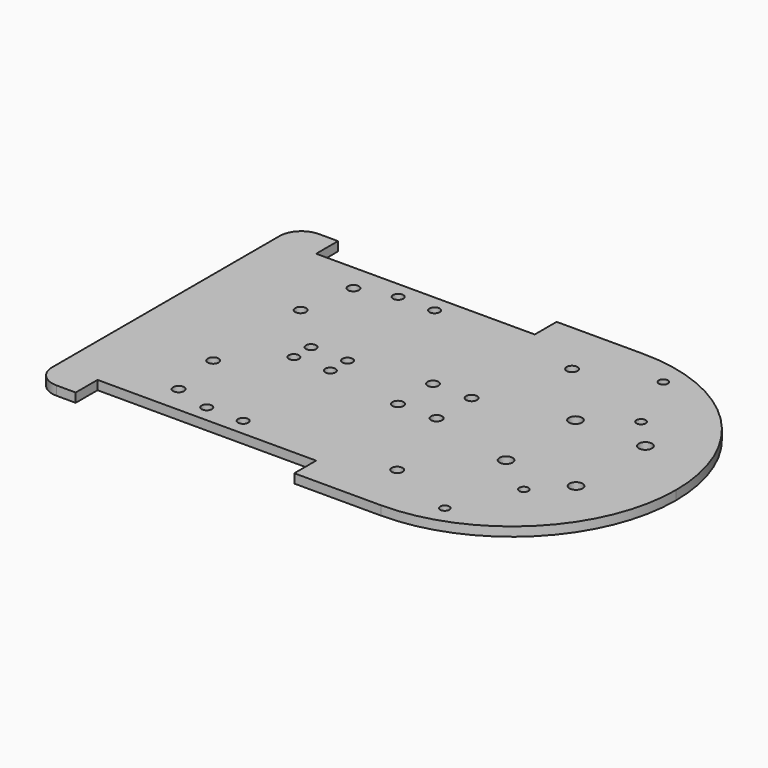
from build123d import *

# Parameters (mm, degrees)
F0_W     = 177.8
F0_H     = 114.3
F1_DEPTH = 3.175
F2_R     = 7.62
F3_W     = 76.2
F3_H     = 9.525
F4_DEPTH = 25.4
F6_D     = 3.556
F8_D     = 3.81
F11_D    = 3.81
F13_D    = 4.572
F15_D    = 3.81
F16_R    = 57.14999
F18_D    = 3.175


# Not quite as in the source:
# - a fillet or chamfer is up to 0.001 mm smaller than in the source, because OpenCascade refuses the exact size


with BuildPart() as f1:
    # F0 (on Top) → F1 (new body)
    with BuildSketch(Plane.XY):
        with Locations((34.6569041669, 50.5347196277)):
            Rectangle(F0_W, F0_H)
    extrude(amount=F1_DEPTH)

    # F2
    f2_edges = [f1.edges().sort_by_distance(p)[0] for p in [
        (-54.243096, 107.68472, 1.5875),
        (-54.243096, -6.61528, 1.5875),
    ]]
    fillet(f2_edges, radius=F2_R)

    # F3 (on face) → F4 (cut)
    with BuildSketch(Plane.XY.offset(3.175)):
        with Locations((-1.8555958331, -1.8527803723)):
            Rectangle(F3_W, F3_H)
        with Locations((-1.8555958331, 102.9222196277)):
            Rectangle(F3_W, F3_H)
    extrude(amount=-F4_DEPTH, mode=Mode.SUBTRACT)

    # F6 (through all)
    with Locations(Plane.XY.offset(3.175)):
        with Locations((-6.6180958331, 8.8279196277), (-6.6180958331, 46.7755196277), (-6.6180958331, 54.2939196277), (-6.6180958331, 92.2415196277), (6.0819041669, 8.8279196277), (6.0819041669, 46.7755196277), (6.0819041669, 54.2939196277), (6.0819041669, 92.2415196277)):
            Hole(F6_D / 2)

    # F8 (through all)
    with Locations(Plane.XY.offset(3.175)):
        with Locations((32.7773041669, 42.9147196277), (46.2393041669, 42.9147196277), (46.2393041669, 58.1547196277), (32.7773041669, 58.1547196277)):
            Hole(F8_D / 2)

    # F11 (through all)
    with Locations(Plane.XY.offset(3.175)):
        with Locations((-22.4930958331, 31.4847196277), (-22.4930958331, 69.5847196277)):
            Hole(F11_D / 2)

    # F13 (through all)
    with Locations(Plane.XY.offset(3.175)):
        with Locations((76.4399041669, 65.6477196277), (76.4399041669, 35.4217196277), (100.8239041669, 35.4217196277), (100.8239041669, 65.6477196277)):
            Hole(F13_D / 2)

    # F15 (through all)
    with Locations(Plane.XY.offset(3.175)):
        with Locations((-19.3180958331, 12.4347196277), (-19.3180958331, 88.6347196277), (56.8819041669, 88.6347196277), (56.8819041669, 12.4347196277)):
            Hole(F15_D / 2)

    # F16 (radius 57.15 in the source; OpenCascade refuses exactly that, so slightly less here)
    f16_edges = [f1.edges().sort_by_distance(p)[0] for p in [
        (123.556904, -6.61528, 1.5875),
        (123.556904, 107.68472, 1.5875),
    ]]
    fillet(f16_edges, radius=F16_R)

    # F18 (through all)
    with Locations(Plane.XY.offset(3.175)):
        with Locations((81.0781642795, 2.9097196277), (90.9841642795, 25.0077196277), (90.9841642795, 76.0617196277), (81.0781642795, 98.1597196277)):
            Hole(F18_D / 2)


solid = f1.part
